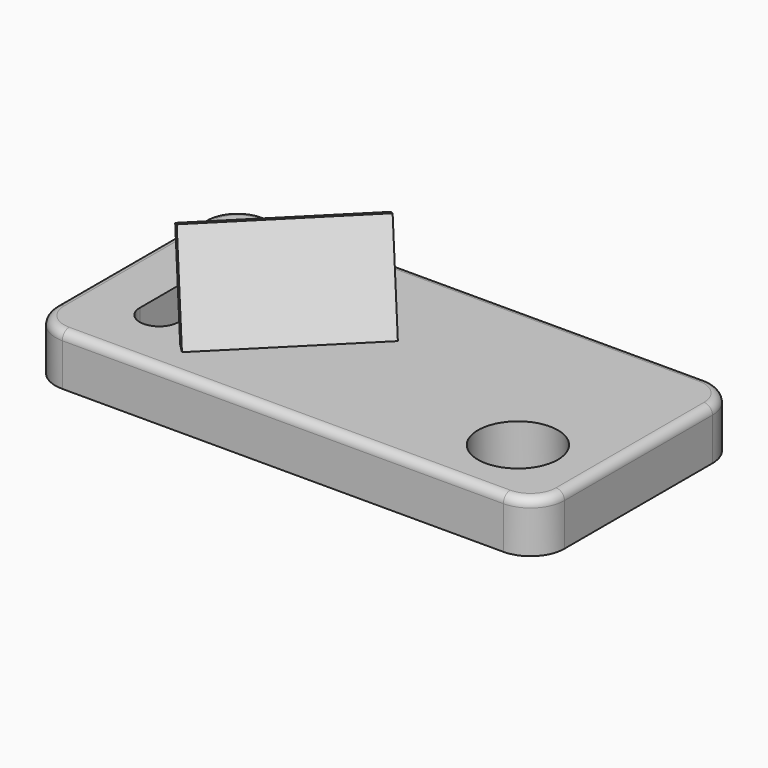
from build123d import *

# Parameters (mm, degrees)
F0_W         = 76.2
F0_H         = 37.856084797
F1_DEPTH     = 7.62
F2_R         = 1.27
F3_T1_DEPTH  = 20.32
F3_T4_ANGLE  = 90
F3_T6_ANGLE  = 90
F3_T8_ANGLE  = 90
F3_T10_ANGLE = 90
F5_DEPTH     = 25.4
F6_R         = 5.9846476777
F7_DEPTH     = 25.4
F10_DEPTH    = 12.7


# Not quite as in the source:
# - a fillet or chamfer that OpenCascade refuses, or shapes differently, is made with other operations: its cross-section is extruded or revolved along the edge and cut away or added


with BuildPart() as f1:
    # F0 (on Top) → F1 (new body)
    with BuildSketch(Plane.XY):
        Rectangle(F0_W, F0_H)
    extrude(amount=F1_DEPTH)

    # F2
    f2_edges = [f1.edges().sort_by_distance(p)[0] for p in [
        (-38.1, 0, 7.62),
        (0, 18.928042, 7.62),
        (38.1, 0, 7.62),
        (0, -18.928042, 7.62),
    ]]
    fillet(f2_edges, radius=F2_R)

    # F3: fillet of radius 5.08 on 4 edges, made by hand

    # F3_s2 → F3_t1 (cut)
    with BuildSketch(Plane.XY.offset(-12.7)):
        with BuildLine():
            ThreePointArc((-33.02, -18.9280423985), (-36.6121024484, -17.4401448469), (-38.1, -13.8480423985))
            Line((-38.1, -13.8480423985), (-38.1, -18.9280423985))
            Line((-38.1, -18.9280423985), (-33.02, -18.9280423985))
        make_face()
        with BuildLine():
            ThreePointArc((-33.02, 18.9280423985), (-36.6121024484, 17.4401448469), (-38.1, 13.8480423985))
            Line((-38.1, 13.8480423985), (-38.1, 18.9280423985))
            Line((-38.1, 18.9280423985), (-33.02, 18.9280423985))
        make_face()
        with BuildLine():
            ThreePointArc((38.1, 13.8480423985), (36.6121024484, 17.4401448469), (33.02, 18.9280423985))
            Line((33.02, 18.9280423985), (38.1, 18.9280423985))
            Line((38.1, 18.9280423985), (38.1, 13.8480423985))
        make_face()
        with BuildLine():
            ThreePointArc((38.1, -13.8480423985), (36.6121024484, -17.4401448469), (33.02, -18.9280423985))
            Line((33.02, -18.9280423985), (38.1, -18.9280423985))
            Line((38.1, -18.9280423985), (38.1, -13.8480423985))
        make_face()
    extrude(amount=F3_T1_DEPTH, mode=Mode.SUBTRACT)

    # F3_s3 → F3_t4 (revolve, cut)
    with BuildSketch(Plane.YZ.offset(33.02)):
        with BuildLine():
            ThreePointArc((-17.6580423985, 7.62), (-18.5560680106, 7.2480256121), (-18.9280423985, 6.35))
            Line((-18.9280423985, 6.35), (-18.9280423985, 7.62))
            Line((-18.9280423985, 7.62), (-17.6580423985, 7.62))
        make_face()
    revolve(axis=Axis((33.02, -13.8480423985, 7.62), (0, 0, 1)), revolution_arc=F3_T4_ANGLE, mode=Mode.SUBTRACT)

    # F3_s5 → F3_t6 (revolve, cut)
    with BuildSketch(Plane.XZ.offset(-13.8480423985)):
        with BuildLine():
            ThreePointArc((36.83, 7.62), (37.7280256121, 7.2480256121), (38.1, 6.35))
            Line((38.1, 6.35), (38.1, 7.62))
            Line((38.1, 7.62), (36.83, 7.62))
        make_face()
    revolve(axis=Axis((33.02, 13.8480423985, 7.62), (0, 0, 1)), revolution_arc=F3_T6_ANGLE, mode=Mode.SUBTRACT)

    # F3_s7 → F3_t8 (revolve, cut)
    with BuildSketch(Plane.YZ.offset(-33.02)):
        with BuildLine():
            ThreePointArc((17.6580423985, 7.62), (18.5560680106, 7.2480256121), (18.9280423985, 6.35))
            Line((18.9280423985, 6.35), (18.9280423985, 7.62))
            Line((18.9280423985, 7.62), (17.6580423985, 7.62))
        make_face()
    revolve(axis=Axis((-33.02, 13.8480423985, 7.62), (0, 0, 1)), revolution_arc=F3_T8_ANGLE, mode=Mode.SUBTRACT)

    # F3_s9 → F3_t10 (revolve, cut)
    with BuildSketch(Plane.XZ.offset(13.8480423985)):
        with BuildLine():
            ThreePointArc((-36.83, 7.62), (-37.7280256121, 7.2480256121), (-38.1, 6.35))
            Line((-38.1, 6.35), (-38.1, 7.62))
            Line((-38.1, 7.62), (-36.83, 7.62))
        make_face()
    revolve(axis=Axis((-33.02, -13.8480423985, 7.62), (0, 0, 1)), revolution_arc=F3_T10_ANGLE, mode=Mode.SUBTRACT)

    # F4 (on face) → F5 (cut)
    with BuildSketch(Plane.XY.offset(7.62)):
        with BuildLine():
            Line((-29.6291131526, 8.6681647226), (-29.6291131526, 0))
            Line((-29.6291131526, 0), (-29.6291131526, -8.6681647226))
            ThreePointArc((-29.6291131526, -8.6681647226), (-26.7311763018, -11.5661015734), (-23.8332394511, -8.6681647226))
            Line((-23.8332394511, -8.6681647226), (-23.8332394511, 0))
            Line((-23.8332394511, 0), (-23.8332394511, 8.6681647226))
            ThreePointArc((-23.8332394511, 8.6681647226), (-26.7311763018, 11.5661015734), (-29.6291131526, 8.6681647226))
        make_face()
    extrude(amount=-F5_DEPTH, mode=Mode.SUBTRACT)

    # F6 (on face) → F7 (cut)
    with BuildSketch(Plane.XY.offset(7.62)):
        with Locations((26.5783518553, -8.1568043679)):
            Circle(F6_R)
    extrude(amount=-F7_DEPTH, mode=Mode.SUBTRACT)

    # F9 (on face) → F10 (join, symmetric)
    with BuildSketch(Plane(origin=(-7.5825373642, -7.5825373642, 0), x_dir=(-0.7071067812, 0.7071067812, 0), z_dir=(0.7071067812, 0.7071067812, 0))):
        Polygon((4.9822961397, 7.62), (10.2810509175, 20.9576525145), (8.66903996, 21.5980688662), (3.1158619095, 7.62), align=None)
    extrude(amount=F10_DEPTH, both=True)


solid = f1.part
